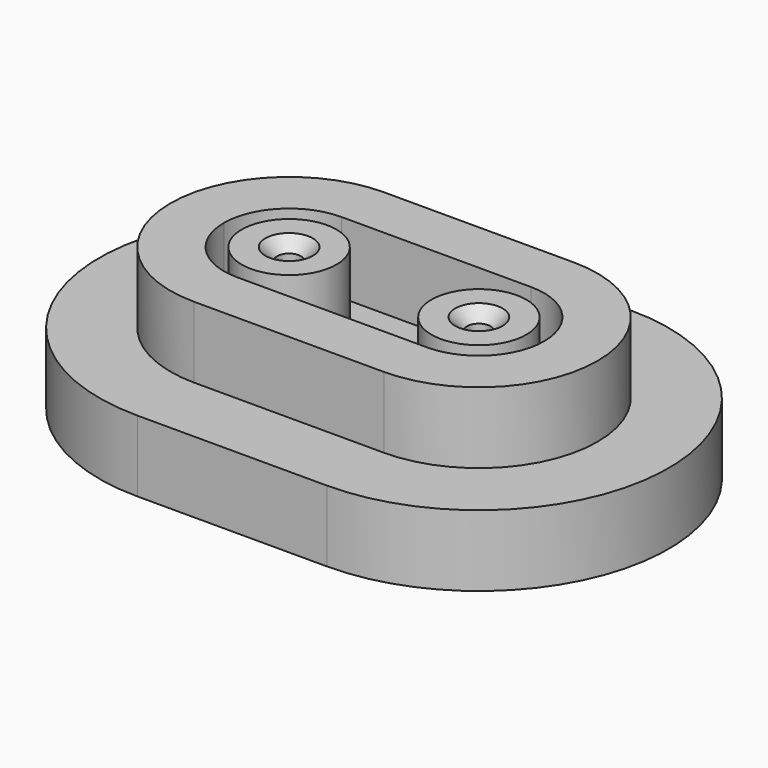
from build123d import *

# Parameters (mm, degrees)
F0_R           = 50.8
F0_R_2         = 12.7
F1_DEPTH       = 76.2
F2_DEPTH       = 152.4
F3_DEPTH       = 152.4
F4_DEPTH       = 25.4
F5_START       = 25.4
F5_DEPTH       = 127
F7_D           = 25.4
F7_CSINK_D     = 50.8
F7_CSINK_ANGLE = 90


# Not quite as in the source:
# - a feature names something its author has since deleted; it is built from what else it names


with BuildPart() as f1:
    # F0 (on Top) → F1 (new body)
    with BuildSketch(Plane.XY):
        with BuildLine():
            ThreePointArc((0, 0), (59.5159020629, -143.6840979371), (203.2, -203.2))
            Line((203.2, -203.2), (406.4, -203.2))
            ThreePointArc((406.4, -203.2), (550.0840979371, -143.6840979371), (609.6, 0))
            ThreePointArc((609.6, 0), (550.0840979371, 143.6840979371), (406.4, 203.2))
            Line((406.4, 203.2), (203.2, 203.2))
            ThreePointArc((203.2, 203.2), (59.5159020629, 143.6840979371), (0, 0))
        make_face()
        with BuildLine():
            Line((406.4, -127), (203.2, -127))
            ThreePointArc((203.2, -127), (113.3974387893, -89.8025612107), (76.2, 0))
            ThreePointArc((76.2, 0), (113.3974387893, 89.8025612107), (203.2, 127))
            Line((203.2, 127), (406.4, 127))
            ThreePointArc((406.4, 127), (496.2025612107, 89.8025612107), (533.4, 0))
            ThreePointArc((533.4, 0), (496.2025612107, -89.8025612107), (406.4, -127))
        make_face(mode=Mode.SUBTRACT)
        with BuildLine():
            ThreePointArc((76.2, 0), (113.3974387893, -89.8025612107), (203.2, -127))
            Line((203.2, -127), (406.4, -127))
            ThreePointArc((406.4, -127), (496.2025612107, -89.8025612107), (533.4, 0))
            ThreePointArc((533.4, 0), (496.2025612107, 89.8025612107), (406.4, 127))
            Line((406.4, 127), (203.2, 127))
            ThreePointArc((203.2, 127), (113.3974387893, 89.8025612107), (76.2, 0))
        make_face()
        with BuildLine():
            Line((406.4, -101.6), (203.2, -101.6))
            ThreePointArc((203.2, -101.6), (131.3579510314, -71.8420489686), (101.6, 0))
            ThreePointArc((101.6, 0), (131.3579510314, 71.8420489686), (203.2, 101.6))
            Line((203.2, 101.6), (406.4, 101.6))
            ThreePointArc((406.4, 101.6), (478.2420489686, 71.8420489686), (508, 0))
            ThreePointArc((508, 0), (478.2420489686, -71.8420489686), (406.4, -101.6))
        make_face(mode=Mode.SUBTRACT)
        with BuildLine():
            ThreePointArc((101.6, 0), (131.3579510314, -71.8420489686), (203.2, -101.6))
            Line((203.2, -101.6), (406.4, -101.6))
            ThreePointArc((406.4, -101.6), (478.2420489686, -71.8420489686), (508, 0))
            ThreePointArc((508, 0), (478.2420489686, 71.8420489686), (406.4, 101.6))
            Line((406.4, 101.6), (203.2, 101.6))
            ThreePointArc((203.2, 101.6), (131.3579510314, 71.8420489686), (101.6, 0))
        make_face()
        with BuildLine():
            ThreePointArc((476.25, 0), (455.7914086659, -49.3914086659), (406.4, -69.85))
            Line((406.4, -69.85), (203.2, -69.85))
            ThreePointArc((203.2, -69.85), (153.8085913341, -49.3914086659), (133.35, 0))
            ThreePointArc((133.35, 0), (153.8085913341, 49.3914086659), (203.2, 69.85))
            Line((203.2, 69.85), (406.4, 69.85))
            ThreePointArc((406.4, 69.85), (455.7914086659, 49.3914086659), (476.25, 0))
        make_face(mode=Mode.SUBTRACT)
        with BuildLine():
            Line((203.2, -69.85), (406.4, -69.85))
            ThreePointArc((406.4, -69.85), (455.7914086659, -49.3914086659), (476.25, 0))
            ThreePointArc((476.25, 0), (455.7914086659, 49.3914086659), (406.4, 69.85))
            Line((406.4, 69.85), (203.2, 69.85))
            ThreePointArc((203.2, 69.85), (153.8085913341, 49.3914086659), (133.35, 0))
            ThreePointArc((133.35, 0), (153.8085913341, -49.3914086659), (203.2, -69.85))
        make_face()
        with Locations((203.2, 0)):
            Circle(F0_R, mode=Mode.SUBTRACT)
        with Locations((406.4, 0)):
            Circle(F0_R, mode=Mode.SUBTRACT)
        with Locations((406.4, 0)):
            Circle(F0_R)
        with Locations((406.4, 0)):
            Circle(F0_R_2, mode=Mode.SUBTRACT)
        with Locations((203.2, 0)):
            Circle(F0_R)
        with Locations((203.2, 0)):
            Circle(F0_R_2, mode=Mode.SUBTRACT)
    extrude(amount=F1_DEPTH)

    # F0 (on Top) → F2 (join)
    with BuildSketch(Plane.XY):
        with BuildLine():
            ThreePointArc((76.2, 0), (113.3974387893, -89.8025612107), (203.2, -127))
            Line((203.2, -127), (406.4, -127))
            ThreePointArc((406.4, -127), (496.2025612107, -89.8025612107), (533.4, 0))
            ThreePointArc((533.4, 0), (496.2025612107, 89.8025612107), (406.4, 127))
            Line((406.4, 127), (203.2, 127))
            ThreePointArc((203.2, 127), (113.3974387893, 89.8025612107), (76.2, 0))
        make_face()
        with BuildLine():
            Line((406.4, -101.6), (203.2, -101.6))
            ThreePointArc((203.2, -101.6), (131.3579510314, -71.8420489686), (101.6, 0))
            ThreePointArc((101.6, 0), (131.3579510314, 71.8420489686), (203.2, 101.6))
            Line((203.2, 101.6), (406.4, 101.6))
            ThreePointArc((406.4, 101.6), (478.2420489686, 71.8420489686), (508, 0))
            ThreePointArc((508, 0), (478.2420489686, -71.8420489686), (406.4, -101.6))
        make_face(mode=Mode.SUBTRACT)
    extrude(amount=F2_DEPTH)

    # F0 (on Top) → F3 (join)
    with BuildSketch(Plane.XY):
        with Locations((203.2, 0)):
            Circle(F0_R)
        with Locations((203.2, 0)):
            Circle(F0_R_2, mode=Mode.SUBTRACT)
        with Locations((406.4, 0)):
            Circle(F0_R)
        with Locations((406.4, 0)):
            Circle(F0_R_2, mode=Mode.SUBTRACT)
        with Locations((203.2, 0)):
            Circle(F0_R_2)
        with Locations((406.4, 0)):
            Circle(F0_R_2)
    extrude(amount=F3_DEPTH)

    # F0 (on Top) → F4 (cut)
    with BuildSketch(Plane.XY):
        with BuildLine():
            ThreePointArc((101.6, 0), (131.3579510314, -71.8420489686), (203.2, -101.6))
            Line((203.2, -101.6), (406.4, -101.6))
            ThreePointArc((406.4, -101.6), (478.2420489686, -71.8420489686), (508, 0))
            ThreePointArc((508, 0), (478.2420489686, 71.8420489686), (406.4, 101.6))
            Line((406.4, 101.6), (203.2, 101.6))
            ThreePointArc((203.2, 101.6), (131.3579510314, 71.8420489686), (101.6, 0))
        make_face()
        with BuildLine():
            ThreePointArc((476.25, 0), (455.7914086659, -49.3914086659), (406.4, -69.85))
            Line((406.4, -69.85), (203.2, -69.85))
            ThreePointArc((203.2, -69.85), (153.8085913341, -49.3914086659), (133.35, 0))
            ThreePointArc((133.35, 0), (153.8085913341, 49.3914086659), (203.2, 69.85))
            Line((203.2, 69.85), (406.4, 69.85))
            ThreePointArc((406.4, 69.85), (455.7914086659, 49.3914086659), (476.25, 0))
        make_face(mode=Mode.SUBTRACT)
        with BuildLine():
            Line((203.2, -69.85), (406.4, -69.85))
            ThreePointArc((406.4, -69.85), (455.7914086659, -49.3914086659), (476.25, 0))
            ThreePointArc((476.25, 0), (455.7914086659, 49.3914086659), (406.4, 69.85))
            Line((406.4, 69.85), (203.2, 69.85))
            ThreePointArc((203.2, 69.85), (153.8085913341, 49.3914086659), (133.35, 0))
            ThreePointArc((133.35, 0), (153.8085913341, -49.3914086659), (203.2, -69.85))
        make_face()
        with Locations((203.2, 0)):
            Circle(F0_R, mode=Mode.SUBTRACT)
        with Locations((406.4, 0)):
            Circle(F0_R, mode=Mode.SUBTRACT)
        with Locations((203.2, 0)):
            Circle(F0_R)
        with Locations((203.2, 0)):
            Circle(F0_R_2, mode=Mode.SUBTRACT)
        with Locations((406.4, 0)):
            Circle(F0_R)
        with Locations((406.4, 0)):
            Circle(F0_R_2, mode=Mode.SUBTRACT)
    extrude(amount=F4_DEPTH, mode=Mode.SUBTRACT)

    # F0 (on Top) → F5 (join)
    with BuildSketch(Plane.XY.offset(F5_START)):
        with BuildLine():
            ThreePointArc((101.6, 0), (131.3579510314, -71.8420489686), (203.2, -101.6))
            Line((203.2, -101.6), (406.4, -101.6))
            ThreePointArc((406.4, -101.6), (478.2420489686, -71.8420489686), (508, 0))
            ThreePointArc((508, 0), (478.2420489686, 71.8420489686), (406.4, 101.6))
            Line((406.4, 101.6), (203.2, 101.6))
            ThreePointArc((203.2, 101.6), (131.3579510314, 71.8420489686), (101.6, 0))
        make_face()
        with BuildLine():
            ThreePointArc((476.25, 0), (455.7914086659, -49.3914086659), (406.4, -69.85))
            Line((406.4, -69.85), (203.2, -69.85))
            ThreePointArc((203.2, -69.85), (153.8085913341, -49.3914086659), (133.35, 0))
            ThreePointArc((133.35, 0), (153.8085913341, 49.3914086659), (203.2, 69.85))
            Line((203.2, 69.85), (406.4, 69.85))
            ThreePointArc((406.4, 69.85), (455.7914086659, 49.3914086659), (476.25, 0))
        make_face(mode=Mode.SUBTRACT)
    extrude(amount=F5_DEPTH)

    # F7 (through all)
    with Locations(Plane.XY.offset(152.4)):
        with Locations((203.2, 0), (406.4, 0)):
            CounterSinkHole(F7_D / 2, F7_CSINK_D / 2, counter_sink_angle=F7_CSINK_ANGLE)


solid = f1.part
